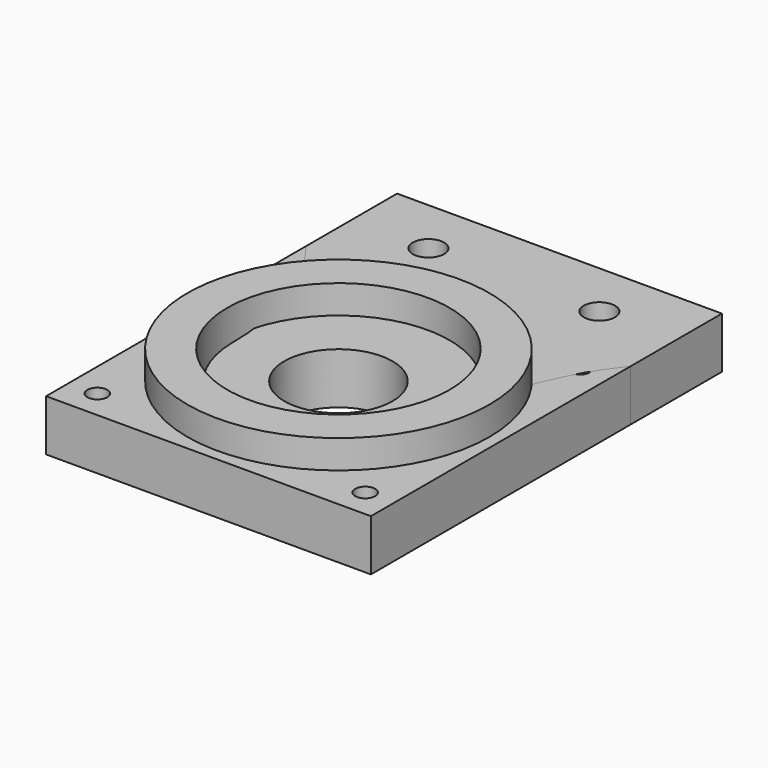
from build123d import *

# Parameters (mm, degrees)
F0_W     = 57
F0_H     = 20
F0_R     = 2.75
F0_H_2   = 57
F0_R_2   = 1.75
F0_R_3   = 19.5
F1_DEPTH = 9
F2_R     = 26.5
F2_R_2   = 19.5
F3_DEPTH = 5
F0_R_4   = 9.5
F4_DEPTH = 9
F6_DEPTH = 9.001


with BuildPart() as f1:
    # F0 (on Top) → F1 (new body)
    with BuildSketch(Plane.XY):
        with Locations((0, 38.5)):
            Rectangle(F0_W, F0_H)
        with Locations((-15, 38.5)):
            Circle(F0_R, mode=Mode.SUBTRACT)
        with Locations((15, 38.5)):
            Circle(F0_R, mode=Mode.SUBTRACT)
        Rectangle(F0_W, F0_H_2)
        with Locations((-23.5, -23.5)):
            Circle(F0_R_2, mode=Mode.SUBTRACT)
        with Locations((23.5, -23.5)):
            Circle(F0_R_2, mode=Mode.SUBTRACT)
        Circle(F0_R_3, mode=Mode.SUBTRACT)
        with Locations((-23.5, 23.5)):
            Circle(F0_R_2, mode=Mode.SUBTRACT)
        with Locations((23.5, 23.5)):
            Circle(F0_R_2, mode=Mode.SUBTRACT)
    extrude(amount=F1_DEPTH)

    # F2 (on face) → F3 (join)
    with BuildSketch(Plane.XY.offset(9)):
        Circle(F2_R)
        Circle(F2_R_2, mode=Mode.SUBTRACT)
    extrude(amount=F3_DEPTH)


with BuildPart() as f4:
    # F0 (on Top) → F4 (new body)
    with BuildSketch(Plane.XY):
        Rectangle(F0_W, F0_H_2)
        with Locations((-23.5, -23.5)):
            Circle(F0_R_2, mode=Mode.SUBTRACT)
        with Locations((23.5, -23.5)):
            Circle(F0_R_2, mode=Mode.SUBTRACT)
        Circle(F0_R_3, mode=Mode.SUBTRACT)
        with Locations((-23.5, 23.5)):
            Circle(F0_R_2, mode=Mode.SUBTRACT)
        with Locations((23.5, 23.5)):
            Circle(F0_R_2, mode=Mode.SUBTRACT)
        Circle(F0_R_3)
        Circle(F0_R_4, mode=Mode.SUBTRACT)
        with Locations((0, 38.5)):
            Rectangle(F0_W, F0_H)
        with Locations((-15, 38.5)):
            Circle(F0_R, mode=Mode.SUBTRACT)
        with Locations((15, 38.5)):
            Circle(F0_R, mode=Mode.SUBTRACT)
        with Locations((23.5, 23.5)):
            Circle(F0_R_2)
        with Locations((-23.5, -23.5)):
            Circle(F0_R_2)
        with Locations((-23.5, 23.5)):
            Circle(F0_R_2)
        with Locations((23.5, -23.5)):
            Circle(F0_R_2)
    extrude(amount=F4_DEPTH)

    # F5 (on face) → F6 (cut, through all)
    with BuildSketch(Plane.XY.offset(9)):
        with BuildLine():
            ThreePointArc((18.5, 0), (0, -18.5), (-18.5, 0))
            ThreePointArc((-18.5, 0), (-21.072545815, 15.1017383105), (-28.5, 28.5))
            Line((-28.5, 28.5), (-28.5, -28.5))
            Line((-28.5, -28.5), (28.5, -28.5))
            Line((28.5, -28.5), (28.5, 28.5))
            ThreePointArc((28.5, 28.5), (21.072545815, 15.1017383105), (18.5, 0))
        make_face()
    extrude(amount=-F6_DEPTH, mode=Mode.SUBTRACT)


solid = Compound([f1.part, f4.part])
